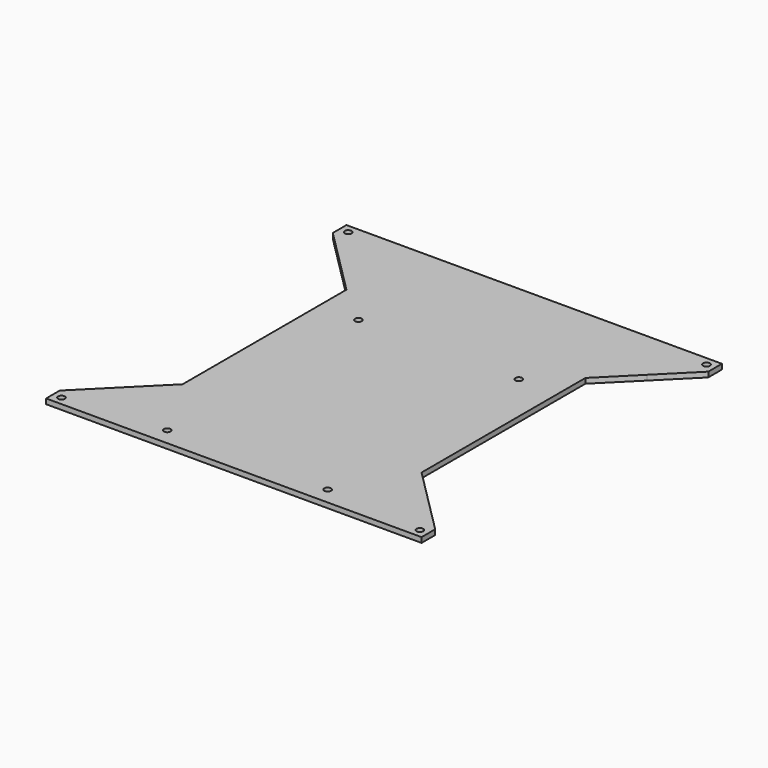
from build123d import *

# Parameters (mm, degrees)
F0_W     = 220
F0_H     = 220
F1_DEPTH = 3
F2_W     = 40
F2_H     = 160
F2_R     = 2
F3_DEPTH = 25
F4_SIZE  = 19.99999
F5_R     = 2
F6_DEPTH = 25


# Not quite as in the source:
# - a fillet or chamfer is up to 0.001 mm smaller than in the source, because OpenCascade refuses the exact size
# - a pattern or mirror of a feature is missing from the dataset's text; its kind, count and spacing are read off the source's solid


with BuildPart() as f1:
    # F0 (on Top) → F1 (new body)
    with BuildSketch(Plane.XY):
        Rectangle(F0_W, F0_H)
    extrude(amount=F1_DEPTH)

    # F2 (on face) → F3 (cut)
    with BuildSketch(Plane.XY.offset(3)):
        with Locations((-90, 0)):
            Rectangle(F2_W, F2_H)
        with Locations((105, 105)):
            Circle(F2_R)
        with Locations((105, -105)):
            Circle(F2_R)
        with Locations((-105, 105)):
            Circle(F2_R)
        with Locations((-105, -105)):
            Circle(F2_R)
    f3 = extrude(amount=-F3_DEPTH, mode=Mode.SUBTRACT)

    # F3_copies: F3 across plane
    add(f3.mirror(Plane(origin=(0, 0, 0), x_dir=(0, 0, 1), z_dir=(1, 0, 0))), mode=Mode.SUBTRACT)

    # F4 (size 20 in the source; OpenCascade refuses exactly that, so slightly less here)
    f4_edges = [f1.edges().sort_by_distance(p)[0] for p in [
        (-110, 80, 1.5),
        (-110, -80, 1.5),
        (-70, -80, 1.5),
        (-70, 80, 1.5),
        (110, 80, 1.5),
        (70, 80, 1.5),
        (70, -80, 1.5),
        (110, -80, 1.5),
    ]]
    chamfer(f4_edges, length=F4_SIZE)

    # F5 (on face) → F6 (cut)
    with BuildSketch(Plane(origin=(0, 0, 0), x_dir=(1, 0, 0), z_dir=(0, 0, -1))):
        with Locations((-47, 100)):
            Circle(F5_R)
        with Locations((-47, -40)):
            Circle(F5_R)
        with Locations((47, -40)):
            Circle(F5_R)
        with Locations((47, 100)):
            Circle(F5_R)
    extrude(amount=-F6_DEPTH, mode=Mode.SUBTRACT)


solid = f1.part
